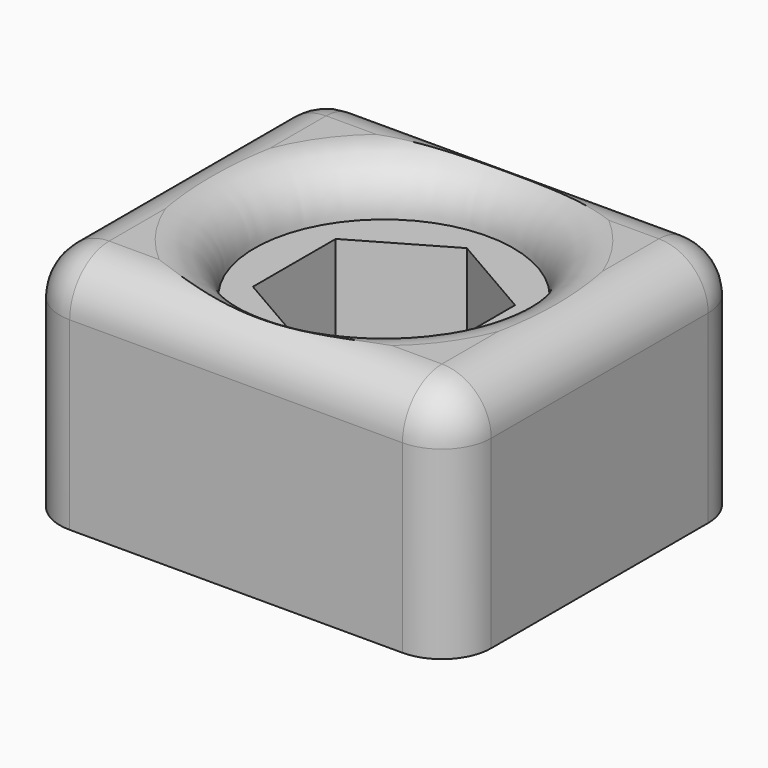
from build123d import *

# Parameters (mm, degrees)
F0_W         = 44.45
F0_H         = 38.1
F1_DEPTH     = 16.51
F3_DEPTH     = 25.4
F4_R         = 13.335
F5_DEPTH     = 5.08
F6_F1_R      = 5.0799
F6_T2_DEPTH  = 69.85
F6_T4_DEPTH  = 69.85
F6_T6_DEPTH  = 27.94
F6_T8_DEPTH  = 24.13
F6_T11_ANGLE = 90
F6_T13_ANGLE = 90
F6_T14_DEPTH = 27.94
F6_T16_DEPTH = 24.13
F6_T19_ANGLE = 90
F6_T21_ANGLE = 90
F8_R         = 6.858
F9_DEPTH     = 7.62


# Not quite as in the source:
# - a fillet or chamfer that OpenCascade refuses, or shapes differently, is made with other operations: its cross-section is extruded or revolved along the edge and cut away or added
# - a fillet or chamfer is up to 0.001 mm smaller than in the source, because OpenCascade refuses the exact size
# - a feature of the source that left no trace in its solid (it failed there, or was rolled back) is left out


with BuildPart() as f1:
    # F0 (on Top) → F1 (new body)
    with BuildSketch(Plane.XY):
        Rectangle(F0_W, F0_H)
    extrude(amount=F1_DEPTH)

    # F2 (on face) → F3 (cut)
    with BuildSketch(Plane.XY.offset(16.51)):
        Polygon((9.2387590076, 5.334), (0, 10.668), (-9.2387590076, 5.334), (-9.2387590076, -5.334), (0, -10.668), (9.2387590076, -5.334), align=None)
    extrude(amount=-F3_DEPTH, mode=Mode.SUBTRACT)

    # F4 (on face) → F5 (cut)
    with BuildSketch(Plane.XY.offset(16.51)):
        Circle(F4_R)
        Polygon((-9.2387590076, 5.334), (0, 10.668), (9.2387590076, 5.334), (9.2387590076, -5.334), (0, -10.668), (-9.2387590076, -5.334), align=None, mode=Mode.SUBTRACT)
    extrude(amount=-F5_DEPTH, mode=Mode.SUBTRACT)

    # F6: fillet of radius 5.08 on 5 edges, made by hand

    # F6_f1 (radius 5.08 in the source; OpenCascade refuses exactly that, so slightly less here)
    f6_f1_edges = [f1.edges().sort_by_distance(p)[0] for p in [
        (-13.335, 0, 16.51),
    ]]
    fillet(f6_f1_edges, radius=F6_F1_R)

    # F6_s3 → F6_t2 (cut)
    with BuildSketch(Plane.YZ.offset(-34.925)):
        with BuildLine():
            ThreePointArc((13.97, 16.51), (17.5621024484, 15.0221024484), (19.05, 11.43))
            Line((19.05, 11.43), (19.1516, 11.43))
            Line((19.1516, 11.43), (19.1516, 16.6116))
            Line((19.1516, 16.6116), (13.97, 16.6116))
            Line((13.97, 16.6116), (13.97, 16.51))
        make_face()
    extrude(amount=F6_T2_DEPTH, mode=Mode.SUBTRACT)

    # F6_s5 → F6_t4 (cut)
    with BuildSketch(Plane.YZ.offset(-34.925)):
        with BuildLine():
            ThreePointArc((-13.97, 16.51), (-17.5621024484, 15.0221024484), (-19.05, 11.43))
            Line((-19.05, 11.43), (-19.1516, 11.43))
            Line((-19.1516, 11.43), (-19.1516, 16.6116))
            Line((-19.1516, 16.6116), (-13.97, 16.6116))
            Line((-13.97, 16.6116), (-13.97, 16.51))
        make_face()
    extrude(amount=F6_T4_DEPTH, mode=Mode.SUBTRACT)

    # F6_s7 → F6_t6 (cut)
    with BuildSketch(Plane.XZ.offset(-13.97)):
        with BuildLine():
            ThreePointArc((17.145, 16.51), (20.7371024484, 15.0221024484), (22.225, 11.43))
            Line((22.225, 11.43), (22.3266, 11.43))
            Line((22.3266, 11.43), (22.3266, 16.6116))
            Line((22.3266, 16.6116), (17.145, 16.6116))
            Line((17.145, 16.6116), (17.145, 16.51))
        make_face()
    extrude(amount=F6_T6_DEPTH, mode=Mode.SUBTRACT)

    # F6_s9 → F6_t8 (cut)
    with BuildSketch(Plane.XY.offset(-12.7)):
        with BuildLine():
            ThreePointArc((22.225, 13.97), (20.7371024484, 17.5621024484), (17.145, 19.05))
            Line((17.145, 19.05), (17.145, 19.1516))
            Line((17.145, 19.1516), (22.3266, 19.1516))
            Line((22.3266, 19.1516), (22.3266, 13.97))
            Line((22.3266, 13.97), (22.225, 13.97))
        make_face()
        with BuildLine():
            ThreePointArc((22.225, -13.97), (20.7371024484, -17.5621024484), (17.145, -19.05))
            Line((17.145, -19.05), (17.145, -19.1516))
            Line((17.145, -19.1516), (22.3266, -19.1516))
            Line((22.3266, -19.1516), (22.3266, -13.97))
            Line((22.3266, -13.97), (22.225, -13.97))
        make_face()
    extrude(amount=F6_T8_DEPTH, mode=Mode.SUBTRACT)

    # F6_s10 → F6_t11 (revolve, cut)
    with BuildSketch(Plane.XY.offset(11.43)):
        with BuildLine():
            ThreePointArc((22.225, -13.97), (20.7371024484, -17.5621024484), (17.145, -19.05))
            Line((17.145, -19.05), (17.145, -19.1516))
            Line((17.145, -19.1516), (22.3266, -19.1516))
            Line((22.3266, -19.1516), (22.3266, -13.97))
            Line((22.3266, -13.97), (22.225, -13.97))
        make_face()
    revolve(axis=Axis((22.225, -13.97, 11.43), (-1, 0, 0)), revolution_arc=F6_T11_ANGLE, mode=Mode.SUBTRACT)

    # F6_s12 → F6_t13 (revolve, cut)
    with BuildSketch(Plane.XY.offset(11.43)):
        with BuildLine():
            ThreePointArc((17.145, 19.05), (20.7371024484, 17.5621024484), (22.225, 13.97))
            Line((22.225, 13.97), (22.3266, 13.97))
            Line((22.3266, 13.97), (22.3266, 19.1516))
            Line((22.3266, 19.1516), (17.145, 19.1516))
            Line((17.145, 19.1516), (17.145, 19.05))
        make_face()
    revolve(axis=Axis((22.225, 13.97, 11.43), (1, 0, 0)), revolution_arc=F6_T13_ANGLE, mode=Mode.SUBTRACT)

    # F6_s15 → F6_t14 (cut)
    with BuildSketch(Plane.XZ.offset(-13.97)):
        with BuildLine():
            ThreePointArc((-17.145, 16.51), (-20.7371024484, 15.0221024484), (-22.225, 11.43))
            Line((-22.225, 11.43), (-22.3266, 11.43))
            Line((-22.3266, 11.43), (-22.3266, 16.6116))
            Line((-22.3266, 16.6116), (-17.145, 16.6116))
            Line((-17.145, 16.6116), (-17.145, 16.51))
        make_face()
    extrude(amount=F6_T14_DEPTH, mode=Mode.SUBTRACT)

    # F6_s17 → F6_t16 (cut)
    with BuildSketch(Plane.XY.offset(-12.7)):
        with BuildLine():
            ThreePointArc((-22.225, -13.97), (-20.7371024484, -17.5621024484), (-17.145, -19.05))
            Line((-17.145, -19.05), (-17.145, -19.1516))
            Line((-17.145, -19.1516), (-22.3266, -19.1516))
            Line((-22.3266, -19.1516), (-22.3266, -13.97))
            Line((-22.3266, -13.97), (-22.225, -13.97))
        make_face()
        with BuildLine():
            ThreePointArc((-17.145, 19.05), (-20.7371024484, 17.5621024484), (-22.225, 13.97))
            Line((-22.225, 13.97), (-22.3266, 13.97))
            Line((-22.3266, 13.97), (-22.3266, 19.1516))
            Line((-22.3266, 19.1516), (-17.145, 19.1516))
            Line((-17.145, 19.1516), (-17.145, 19.05))
        make_face()
    extrude(amount=F6_T16_DEPTH, mode=Mode.SUBTRACT)

    # F6_s18 → F6_t19 (revolve, cut)
    with BuildSketch(Plane.XY.offset(11.43)):
        with BuildLine():
            ThreePointArc((-17.145, 19.05), (-20.7371024484, 17.5621024484), (-22.225, 13.97))
            Line((-22.225, 13.97), (-22.3266, 13.97))
            Line((-22.3266, 13.97), (-22.3266, 19.1516))
            Line((-22.3266, 19.1516), (-17.145, 19.1516))
            Line((-17.145, 19.1516), (-17.145, 19.05))
        make_face()
    revolve(axis=Axis((-22.225, 13.97, 11.43), (1, 0, 0)), revolution_arc=F6_T19_ANGLE, mode=Mode.SUBTRACT)

    # F6_s20 → F6_t21 (revolve, cut)
    with BuildSketch(Plane.XY.offset(11.43)):
        with BuildLine():
            ThreePointArc((-17.145, -19.05), (-20.7371024484, -17.5621024484), (-22.225, -13.97))
            Line((-22.225, -13.97), (-22.3266, -13.97))
            Line((-22.3266, -13.97), (-22.3266, -19.1516))
            Line((-22.3266, -19.1516), (-17.145, -19.1516))
            Line((-17.145, -19.1516), (-17.145, -19.05))
        make_face()
    revolve(axis=Axis((-22.225, -13.97, 11.43), (-1, 0, 0)), revolution_arc=F6_T21_ANGLE, mode=Mode.SUBTRACT)

    # F8 (on face) → F9 (join)
    with BuildSketch(Plane(origin=(0, 0, 0), x_dir=(1, 0, 0), z_dir=(0, 0, -1))):
        with BuildLine():
            Line((-17.145, -19.05), (17.145, -19.05))
            ThreePointArc((17.145, -19.05), (20.7371024484, -17.5621024484), (22.225, -13.97))
            Line((22.225, -13.97), (22.225, 13.97))
            ThreePointArc((22.225, 13.97), (20.7371024484, 17.5621024484), (17.145, 19.05))
            Line((17.145, 19.05), (-17.145, 19.05))
            ThreePointArc((-17.145, 19.05), (-20.7371024484, 17.5621024484), (-22.225, 13.97))
            Line((-22.225, 13.97), (-22.225, -13.97))
            ThreePointArc((-22.225, -13.97), (-20.7371024484, -17.5621024484), (-17.145, -19.05))
        make_face()
        Polygon((9.2387590076, 5.334), (9.2387590076, -5.334), (0, -10.668), (-9.2387590076, -5.334), (-9.2387590076, 5.334), (0, 10.668), align=None, mode=Mode.SUBTRACT)
        Polygon((0, -10.668), (9.2387590076, -5.334), (9.2387590076, 5.334), (0, 10.668), (-9.2387590076, 5.334), (-9.2387590076, -5.334), align=None)
        Circle(F8_R, mode=Mode.SUBTRACT)
    extrude(amount=F9_DEPTH)


solid = f1.part
